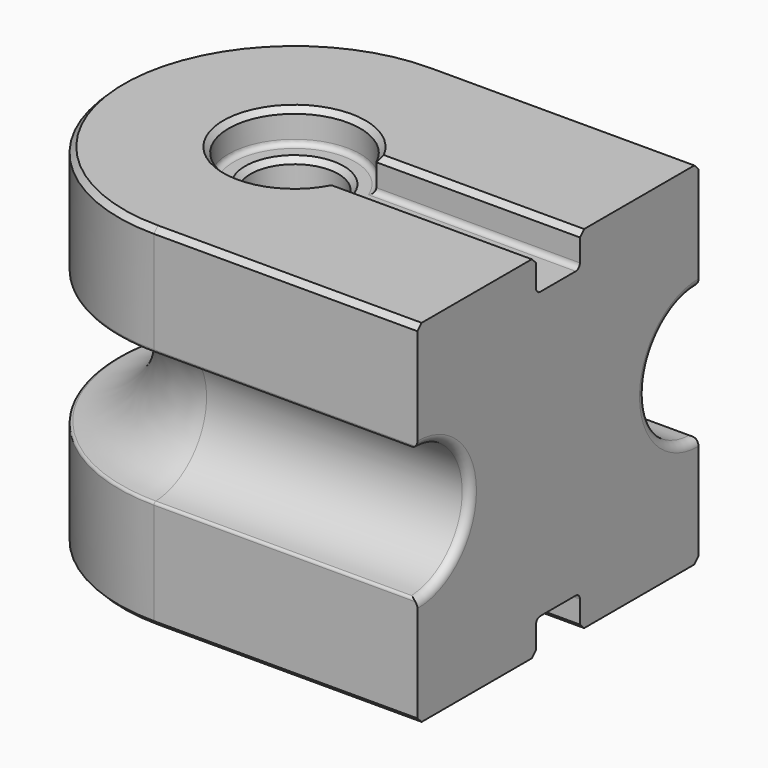
from build123d import *

# Parameters (mm, degrees)
F1_DEPTH     = 50.8
F4_R         = 19.05
F6_R         = 12.7
F7_DEPTH     = 101.6010001
F8_R         = 19.05
F9_DEPTH     = 9.525
F10_R        = 19.05
F11_DEPTH    = 9.525
F12_SIZE     = 1.524
F13_R        = 0.762
F14_T2_ANGLE = 210.0216204264
F14_T4_ANGLE = 210.0216204264
F15_W        = 76.2
F15_H        = 15.875
F16_DEPTH    = 9.525
F17_W        = 76.2
F17_H        = 15.875
F18_DEPTH    = 9.525
F19_SIZE     = 1.524
F20_R        = 1.524


# Not quite as in the source:
# - a fillet or chamfer that OpenCascade refuses, or shapes differently, is made with other operations: its cross-section is extruded or revolved along the edge and cut away or added


with BuildPart() as f1:
    # F0 (on Top) → F1 (new body, symmetric)
    with BuildSketch(Plane.XY):
        with BuildLine():
            Line((76.2, 50.8), (0, 50.8))
            ThreePointArc((0, 50.8), (-50.8, 0), (0, -50.8))
            Line((0, -50.8), (76.2, -50.8))
            Line((76.2, -50.8), (76.2, 50.8))
        make_face()
    extrude(amount=F1_DEPTH, both=True)

    # F5: sweep along a path in F2
    with BuildLine(Plane.XY) as f5_path:
        Line((88.8873545716, 50.8), (-0.0126454284, 50.8))
        ThreePointArc((-0.0126454284, 50.8), (-50.8126454284, 0), (-0.0126454284, -50.8))
        Line((-0.0126454284, -50.8), (88.8873545716, -50.8))
    # F4 (on line) → F5 (sweep, cut)
    with BuildSketch(Plane.YZ.offset(88.8873545716)):
        with Locations((50.8, 0)):
            Circle(F4_R)
    sweep(path=f5_path.line, mode=Mode.SUBTRACT)

    # F6 (on face) → F7 (cut, through all)
    with BuildSketch(Plane.XY.offset(50.8)):
        Circle(F6_R)
    extrude(amount=-F7_DEPTH, mode=Mode.SUBTRACT)

    # F8 (on face) → F9 (cut)
    with BuildSketch(Plane.XY.offset(50.8)):
        Circle(F8_R)
    extrude(amount=-F9_DEPTH, mode=Mode.SUBTRACT)

    # F10 (on face) → F11 (cut)
    with BuildSketch(Plane(origin=(0, 0, -50.8), x_dir=(1, 0, 0), z_dir=(0, 0, -1))):
        Circle(F10_R)
    extrude(amount=-F11_DEPTH, mode=Mode.SUBTRACT)

    # F12
    f12_edges = [f1.edges().sort_by_distance(p)[0] for p in [
        (38.1, -50.8, 50.8),
        (38.1, 50.8, -50.8),
    ]]
    chamfer(f12_edges, length=F12_SIZE)

    # F13
    f13_edges = [f1.edges().sort_by_distance(p)[0] for p in [
        (38.1, -50.8, -19.05),
        (38.1, -50.8, 19.05),
        (-0.006323, 50.799999, -19.05),
        (-50.8, 0, -19.049996),
        (-0.006323, -50.799999, -19.05),
        (-0.006323, -50.799999, 19.05),
        (38.1, 50.8, -19.05),
        (-0.006323, 50.799999, 19.05),
        (38.1, 50.8, 19.05),
        (-50.8, 0, 19.049996),
    ]]
    fillet(f13_edges, radius=F13_R)

    # F14: fillet of radius 2.286 on 2 edges, made by hand

    # F14_s1 → F14_t2 (revolve, cut)
    with BuildSketch(Plane(origin=(0, 47.3922513753, 12.7082996284), x_dir=(1, 0, 0), z_dir=(0, 0.9658769767, 0.2590012854))):
        with BuildLine():
            ThreePointArc((76.2, 34.4932652985), (75.5304461018, 32.8768191967), (73.914, 32.2072652985))
            Line((73.914, 32.2072652985), (76.2, 32.2072652985))
            Line((76.2, 32.2072652985), (76.2, 34.4932652985))
        make_face()
    revolve(axis=Axis((76.2, 50.8, 0), (-1, 0, 0)), revolution_arc=F14_T2_ANGLE, mode=Mode.SUBTRACT)

    # F14_s3 → F14_t4 (revolve, cut)
    with BuildSketch(Plane(origin=(0, -47.3922513753, 12.7082996284), x_dir=(1, 0, 0), z_dir=(0, -0.9658769767, 0.2590012854))):
        with BuildLine():
            ThreePointArc((76.2, -34.4932652985), (75.5304461018, -32.8768191967), (73.914, -32.2072652985))
            Line((73.914, -32.2072652985), (76.2, -32.2072652985))
            Line((76.2, -32.2072652985), (76.2, -34.4932652985))
        make_face()
    revolve(axis=Axis((76.2, -50.8, 0), (1, 0, 0)), revolution_arc=F14_T4_ANGLE, mode=Mode.SUBTRACT)

    # F15 (on face) → F16 (cut)
    with BuildSketch(Plane(origin=(0, 0, -50.8), x_dir=(1, 0, 0), z_dir=(0, 0, -1))):
        with Locations((38.1, 0)):
            Rectangle(F15_W, F15_H)
    extrude(amount=-F16_DEPTH, mode=Mode.SUBTRACT)

    # F17 (on face) → F18 (cut)
    with BuildSketch(Plane.XY.offset(50.8)):
        with Locations((38.1, 0)):
            Rectangle(F17_W, F17_H)
    extrude(amount=-F18_DEPTH, mode=Mode.SUBTRACT)

    # F19
    f19_edges = [f1.edges().sort_by_distance(p)[0] for p in [
        (-19.05, 0, 50.8),
        (46.75879, 7.9375, 50.8),
        (46.75879, -7.9375, 50.8),
        (-12.7, 0, 41.275),
        (-19.05, 0, -50.8),
        (-12.7, 0, -41.275),
        (46.75879, -7.9375, -50.8),
        (46.75879, 7.9375, -50.8),
    ]]
    chamfer(f19_edges, length=F19_SIZE)

    # F20
    f20_edges = [f1.edges().sort_by_distance(p)[0] for p in [
        (-19.05, 0, -41.275),
        (46.75879, -7.9375, -41.275),
        (46.75879, 7.9375, -41.275),
        (-19.05, 0, 41.275),
        (46.75879, 7.9375, 41.275),
        (46.75879, -7.9375, 41.275),
    ]]
    fillet(f20_edges, radius=F20_R)


solid = f1.part
